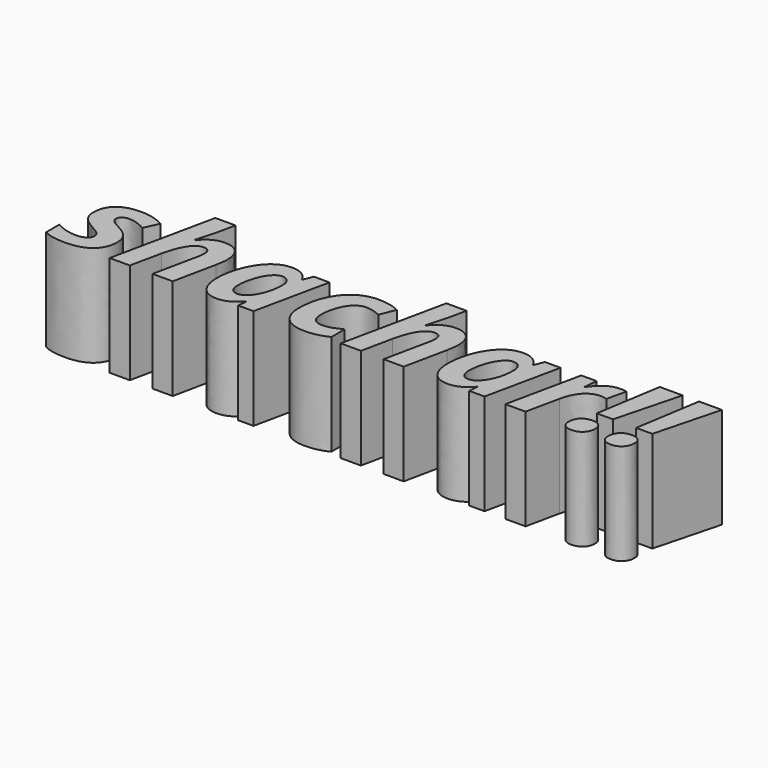
from build123d import *

# Parameters (mm, degrees)
F0_TEXT_SIZE = 34.0054189099
F1_DEPTH     = 25


# Not quite as in the source:
# - Text() gives the source's letters only with a copy of the font that has no kerning and outlines rounded to 1/6400 em; it was checked with that copy


with BuildPart() as f1:
    # F0 (on Top) → F1 (new body)
    with BuildSketch(Plane.XY):
        with Locations((-74.8814249753, -10.5441622237)):
            Text('shachar!!', F0_TEXT_SIZE, font='Open Sans', font_style=FontStyle.BOLDITALIC, text_align=(TextAlign.LEFT, TextAlign.BOTTOM))
    extrude(amount=F1_DEPTH)


solid = f1.part
